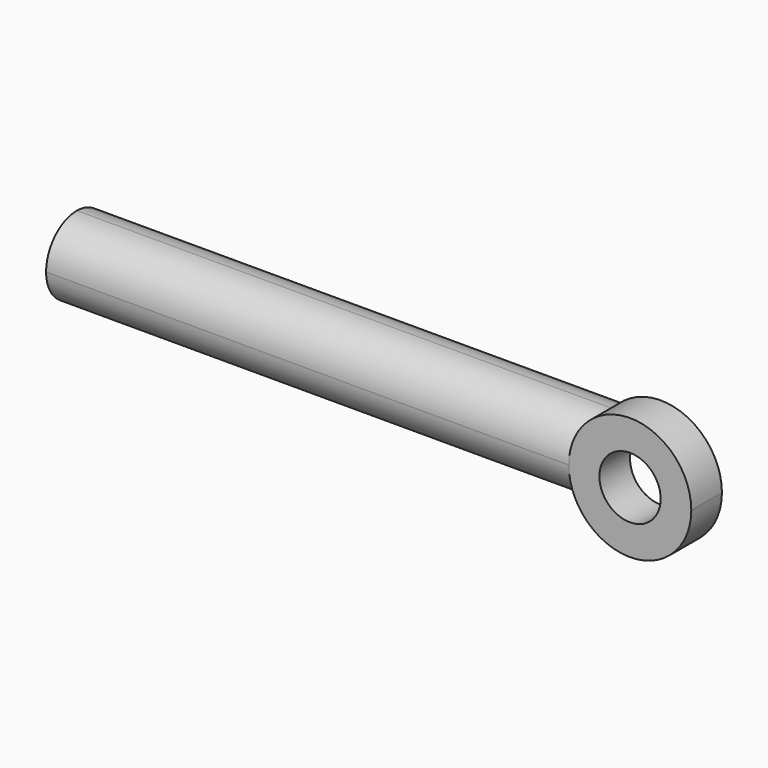
from build123d import *

# Parameters (mm, degrees)
F1_DEPTH = 6.35
F2_R     = 6.3499
F0_R     = 5.08
F3_DEPTH = 6.35


# Not quite as in the source:
# - a fillet or chamfer is up to 0.001 mm smaller than in the source, because OpenCascade refuses the exact size


with BuildPart() as f1:
    # F0 (on Front) → F1 (new body, symmetric)
    with BuildSketch(Plane.XZ):
        with BuildLine():
            Line((44.45, 6.35), (-44.45, 6.35))
            ThreePointArc((-44.45, 6.35), (-42.7945407024, 3.3649028089), (-42.221147458, 0))
            ThreePointArc((-42.221147458, 0), (-42.7945407024, -3.3649028089), (-44.45, -6.35))
            Line((-44.45, -6.35), (44.45, -6.35))
            ThreePointArc((44.45, -6.35), (42.221147458, 0), (44.45, 6.35))
        make_face()
        with BuildLine():
            ThreePointArc((-42.221147458, 0), (-42.7945407024, 3.3649028089), (-44.45, 6.35))
            Line((-44.45, 6.35), (-44.45, -6.35))
            ThreePointArc((-44.45, -6.35), (-42.7945407024, -3.3649028089), (-42.221147458, 0))
        make_face()
    extrude(amount=F1_DEPTH, both=True)

    # F2 (radius 6.35 in the source; OpenCascade refuses exactly that, so slightly less here)
    f2_edges = [f1.edges().sort_by_distance(p)[0] for p in [
        (0, -6.35, 6.35),
        (0, 6.35, 6.35),
        (0, -6.35, -6.35),
        (0, 6.35, -6.35),
    ]]
    fillet(f2_edges, radius=F2_R)

    # F0 (on Front) → F3 (join)
    with BuildSketch(Plane.XZ):
        with BuildLine():
            ThreePointArc((62.541147458, 0), (55.7460502669, 9.5866067556), (44.45, 6.35))
            Line((44.45, 6.35), (44.45, -6.35))
            ThreePointArc((44.45, -6.35), (55.7460502669, -9.5866067556), (62.541147458, 0))
        make_face()
        with Locations((52.381147458, 0)):
            Circle(F0_R, mode=Mode.SUBTRACT)
        with BuildLine():
            Line((44.45, -6.35), (44.45, 6.35))
            ThreePointArc((44.45, 6.35), (42.221147458, 0), (44.45, -6.35))
        make_face()
    extrude(amount=F3_DEPTH)


solid = f1.part
